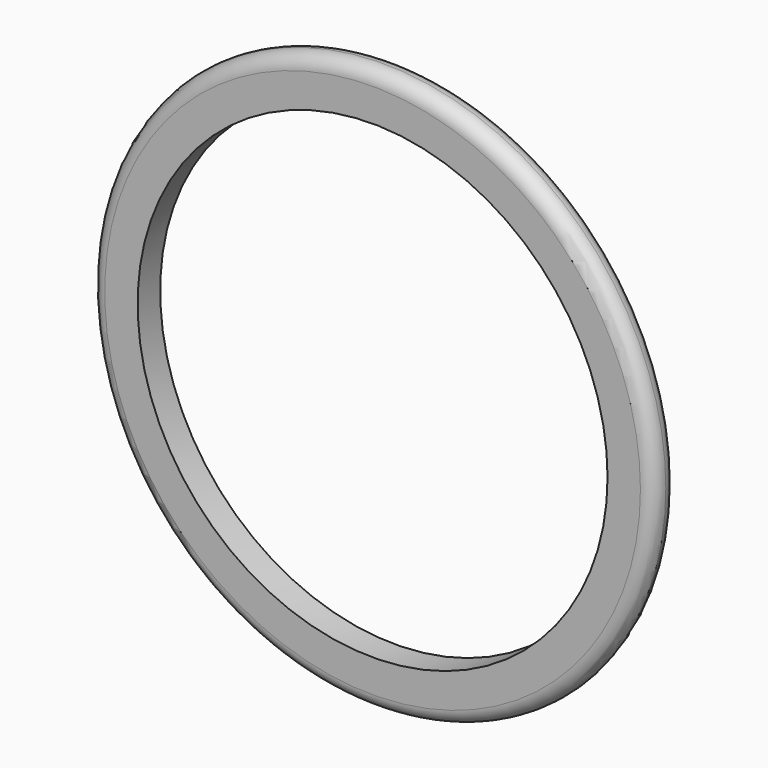
from build123d import *

# Parameters (mm, degrees)
F0_R     = 300
F0_R_2   = 250
F1_DEPTH = 30
F2_R     = 14.99999


# Not quite as in the source:
# - a fillet or chamfer is up to 0.001 mm smaller than in the source, because OpenCascade refuses the exact size


with BuildPart() as f1:
    # F0 (on Front) → F1 (new body)
    with BuildSketch(Plane.XZ):
        Circle(F0_R)
        Circle(F0_R_2, mode=Mode.SUBTRACT)
    extrude(amount=F1_DEPTH)

    # F2 (radius 15 in the source; OpenCascade refuses exactly that, so slightly less here)
    f2_edges = [f1.edges().sort_by_distance(p)[0] for p in [
        (300, -15, 0),
        (-300, 0, 0),
        (-300, -30, 0),
    ]]
    fillet(f2_edges, radius=F2_R)


solid = f1.part
